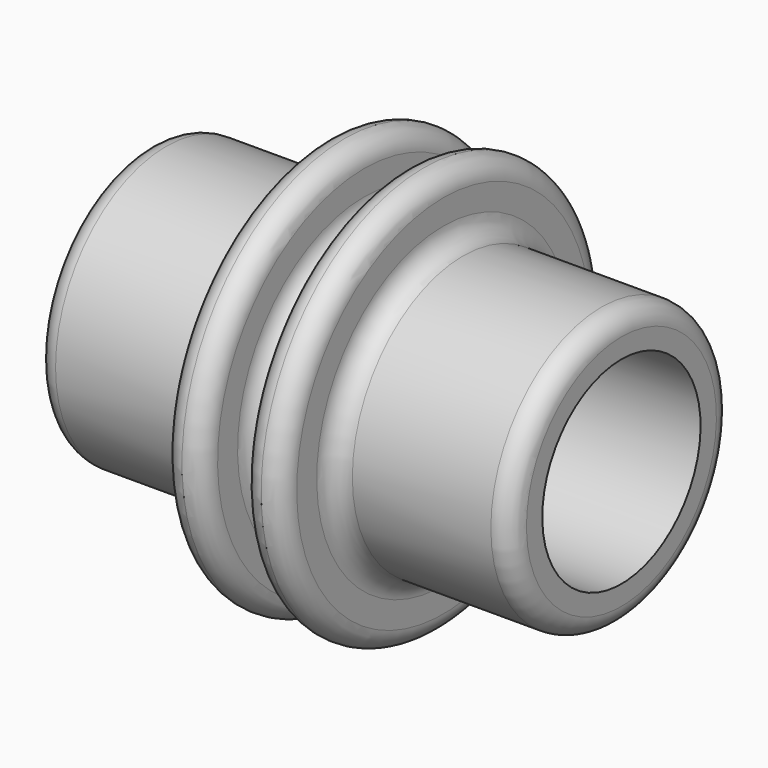
from build123d import *

# Parameters (mm, degrees)
F4_R = 0.79374


# Not quite as in the source:
# - a fillet or chamfer is up to 0.001 mm smaller than in the source, because OpenCascade refuses the exact size


with BuildPart() as f2:
    # F0 (on Front) → F2 (revolve)
    with BuildSketch(Plane.XZ):
        Polygon((0, 5.55625), (0, 3.96875), (9.525, 3.96875), (9.525, 5.55625), (2.38125, 5.55625), (2.38125, 8.1463824849), (0.79375, 8.1463824849), (0.79375, 5.55625), align=None)
    revolve(axis=Axis((1.0093955789, 0, 0), (1, 0, 0)))

    # F3: F2 across face


with BuildPart() as f2_1:
    add(f2.part)
    add(f2.part.mirror(Plane(origin=(0, 0, 0), x_dir=(0, -1, 0), z_dir=(-1, 0, 0))))

    # F4 (radius 0.79375 in the source; OpenCascade refuses exactly that, so slightly less here)
    f4_edges = [f2_1.edges().sort_by_distance(p)[0] for p in [
        (-0.79375, 0, -8.146382),
        (-2.38125, 0, -8.146382),
        (-9.525, 0, -5.55625),
        (-2.38125, 0, -5.55625),
        (-0.79375, 0, -5.55625),
        (2.38125, 0, -8.146382),
        (0.79375, 0, -8.146382),
        (0.79375, 0, -5.55625),
        (2.38125, 0, -5.55625),
        (9.525, 0, -5.55625),
    ]]
    fillet(f4_edges, radius=F4_R)


solid = f2_1.part
